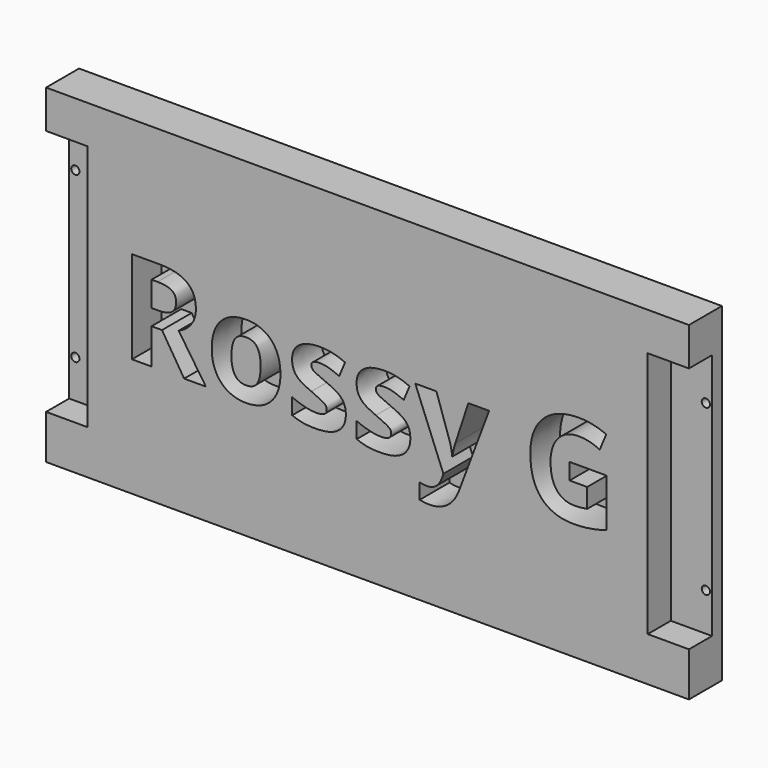
from build123d import *

# Parameters (mm, degrees)
F0_W         = 198.12
F0_H         = 101.6
F1_DEPTH     = 12.7
F2_R         = 1.27
F3_DEPTH     = 3.81
F4_TEXT_SIZE = 39.9885203559
F5_DEPTH     = 11.43
F6_W         = 12.7
F6_H         = 76.2
F7_DEPTH     = 8.89


# Not quite as in the source:
# - Text() gives the source's letters only with a copy of the font that has no kerning and outlines rounded to 1/6400 em; it was checked with that copy


with BuildPart() as f1:
    # F0 (on Front) → F1 (new body)
    with BuildSketch(Plane.XZ):
        Rectangle(F0_W, F0_H)
    extrude(amount=F1_DEPTH)

    # F2 (on Front) → F3 (cut)
    with BuildSketch(Plane.XZ):
        with Locations((-97.155, 25.4)):
            Circle(F2_R)
        with Locations((-97.155, -25.4)):
            Circle(F2_R)
        with Locations((97.155, 25.4)):
            Circle(F2_R)
        with Locations((97.155, -25.4)):
            Circle(F2_R)
    extrude(amount=F3_DEPTH, mode=Mode.SUBTRACT)

    # F4 (on face) → F5 (cut)
    with BuildSketch(Plane.XZ.offset(12.7)):
        with Locations((-76.2, -14.3351781088)):
            Text('Rossy G', F4_TEXT_SIZE, font='Open Sans', font_style=FontStyle.BOLD, text_align=(TextAlign.LEFT, TextAlign.BOTTOM))
    extrude(amount=-F5_DEPTH, mode=Mode.SUBTRACT)

    # F6 (on face) → F7 (cut)
    with BuildSketch(Plane.XZ.offset(12.7)):
        with Locations((-92.71, 0.914733386)):
            Rectangle(F6_W, F6_H)
        with Locations((92.71, 0.914733386)):
            Rectangle(F6_W, F6_H)
    extrude(amount=-F7_DEPTH, mode=Mode.SUBTRACT)


solid = f1.part
